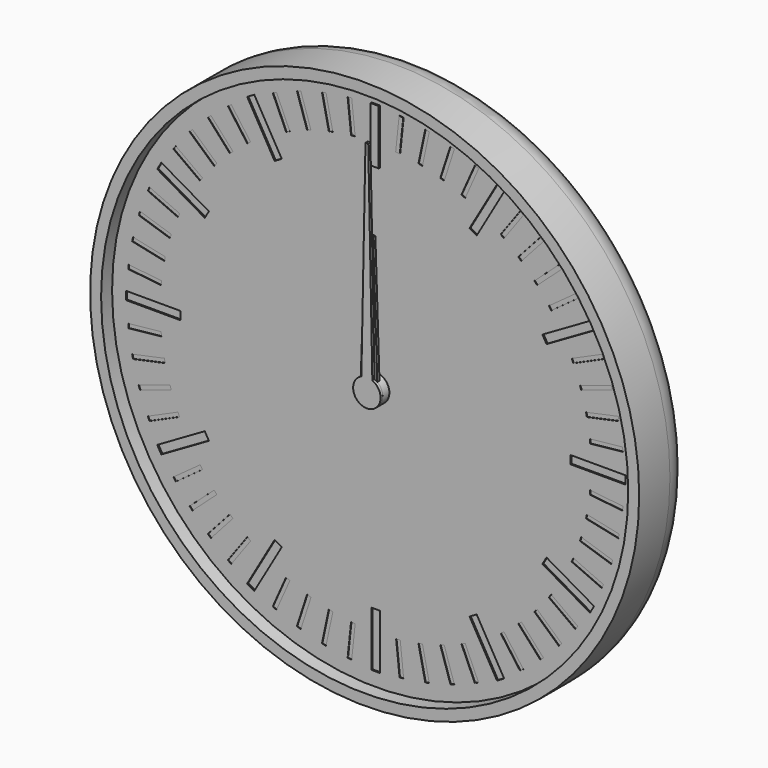
from build123d import *

# Parameters (mm, degrees)
F0_R      = 100
F1_DEPTH  = 24
F2_R      = 10
F3_T      = -4
F4_R      = 5
F4_R_2    = 3
F5_DEPTH  = 2
F6_DEPTH  = 19
F7_DEPTH  = 8
F9_DEPTH  = 4
F11_DEPTH = 4
F12_R     = 5
F12_R_2   = 3
F13_DEPTH = 2
F14_R     = 3
F15_DEPTH = 4
F17_DEPTH = 4
F18_R     = 3
F19_DEPTH = 2
F20_R     = 98
F20_R_2   = 5
F21_DEPTH = 1
F23_R     = 5
F23_R_2   = 3
F24_DEPTH = 2
F25_W     = 3
F25_H     = 20
F25_W_2   = 20
F25_H_2   = 3
F26_DEPTH = 0.5
F27_W     = 1.5
F27_H     = 12
F27_W_2   = 12
F27_H_2   = 1.5
F28_DEPTH = 0.2
F29_DEPTH = 1
F30_DEPTH = 0.4
F31_R     = 5
F31_R_2   = 3
F32_DEPTH = 5
F33_R     = 3
F34_DEPTH = 1
F36_DEPTH = 1


with BuildPart() as f1:
    # F0 (on Front) → F1 (new body)
    with BuildSketch(Plane.XZ):
        Circle(F0_R)
    extrude(amount=F1_DEPTH)

    # F2
    f2_edges = [f1.edges().sort_by_distance(p)[0] for p in [
        (-100, 0, 0),
    ]]
    fillet(f2_edges, radius=F2_R)

    # F3
    f3_openings = [f1.faces().sort_by_distance(p)[0] for p in [
        (0, -24, 0),
    ]]
    offset(amount=F3_T, openings=f3_openings)

    # F4 (on face) → F5 (join)
    with BuildSketch(Plane.XZ.offset(4)):
        Circle(F4_R)
        Circle(F4_R_2, mode=Mode.SUBTRACT)
        with Locations((40, 0)):
            Circle(F4_R)
        with Locations((40, 0)):
            Circle(F4_R_2, mode=Mode.SUBTRACT)
    extrude(amount=F5_DEPTH)


with BuildPart() as f6:
    # F6 (new): a face of the model
    f6_faces = [f1.part.faces().sort_by_distance(p)[0] for p in [
        (0, -4, 0),
    ]]
    extrude(f6_faces, amount=F6_DEPTH)

    # F8 (on face) → F9 (join)
    with BuildSketch(Plane.XZ.offset(6)):
        with BuildLine():
            ThreePointArc((9.2729637667, -1.3794085621), (9.3494561423, -0.6915886375), (9.375, 0))
            ThreePointArc((9.375, 0), (9.3494561423, 0.6915886375), (9.2729637667, 1.3794085621))
            ThreePointArc((9.2729637667, 1.3794085621), (8.9161548403, 2.8970343223), (8.3127812852, 4.3345463782))
            ThreePointArc((8.3127812852, 4.3345463782), (7.5845343223, 5.5104867402), (6.6911892658, 6.566476316))
            ThreePointArc((6.6911892658, 6.566476316), (5.5104867402, 7.5845343223), (4.1773988938, 8.3928519278))
            ThreePointArc((4.1773988938, 8.3928519278), (2.8970343223, 8.9161548403), (1.5536078905, 9.2453733036))
            ThreePointArc((1.5536078905, 9.2453733036), (0, 9.375), (-1.5536078905, 9.2453733036))
            ThreePointArc((-1.5536078905, 9.2453733036), (-2.8970343223, 8.9161548403), (-4.1773988938, 8.3928519278))
            ThreePointArc((-4.1773988938, 8.3928519278), (-5.5104867402, 7.5845343223), (-6.6911892658, 6.566476316))
            ThreePointArc((-6.6911892658, 6.566476316), (-7.5845343223, 5.5104867402), (-8.3127812852, 4.3345463782))
            ThreePointArc((-8.3127812852, 4.3345463782), (-8.9161548403, 2.8970343223), (-9.2729637667, 1.3794085621))
            ThreePointArc((-9.2729637667, 1.3794085621), (-9.375, 0), (-9.2729637667, -1.3794085621))
            ThreePointArc((-9.2729637667, -1.3794085621), (-8.9161548403, -2.8970343223), (-8.3127812852, -4.3345463782))
            ThreePointArc((-8.3127812852, -4.3345463782), (-7.5845343223, -5.5104867402), (-6.6911892658, -6.566476316))
            ThreePointArc((-6.6911892658, -6.566476316), (-5.5104867402, -7.5845343223), (-4.1773988938, -8.3928519278))
            ThreePointArc((-4.1773988938, -8.3928519278), (-2.8970343223, -8.9161548403), (-1.5536078905, -9.2453733036))
            ThreePointArc((-1.5536078905, -9.2453733036), (0, -9.375), (1.5536078905, -9.2453733036))
            ThreePointArc((1.5536078905, -9.2453733036), (2.8970343223, -8.9161548403), (4.1773988938, -8.3928519278))
            ThreePointArc((4.1773988938, -8.3928519278), (5.5104867402, -7.5845343223), (6.6911892658, -6.566476316))
            ThreePointArc((6.6911892658, -6.566476316), (7.5845343223, -5.5104867402), (8.3127812852, -4.3345463782))
            ThreePointArc((8.3127812852, -4.3345463782), (8.9161548403, -2.8970343223), (9.2729637667, -1.3794085621))
        make_face()
        with BuildLine():
            ThreePointArc((8.3127812852, 4.3345463782), (8.9161548403, 2.8970343223), (9.2729637667, 1.3794085621))
            Line((9.2729637667, 1.3794085621), (11.1823199426, 2.3946312492))
            Line((11.1823199426, 2.3946312492), (10.8182678729, 3.515068311))
            Line((10.8182678729, 3.515068311), (10.4542158031, 4.6355053728))
            Line((10.4542158031, 4.6355053728), (8.3127812852, 4.3345463782))
        make_face()
        with BuildLine():
            Line((11.1823199426, -2.3946312492), (9.2729637667, -1.3794085621))
            ThreePointArc((9.2729637667, -1.3794085621), (8.9161548403, -2.8970343223), (8.3127812852, -4.3345463782))
            Line((8.3127812852, -4.3345463782), (10.4542158031, -4.6355053728))
            Line((10.4542158031, -4.6355053728), (10.8182678729, -3.515068311))
            Line((10.8182678729, -3.515068311), (11.1823199426, -2.3946312492))
        make_face()
        with BuildLine():
            ThreePointArc((4.1773988938, 8.3928519278), (5.5104867402, 7.5845343223), (6.6911892658, 6.566476316))
            Line((6.6911892658, 6.566476316), (7.6391579371, 8.5101001246))
            Line((7.6391579371, 8.5101001246), (6.6860572448, 9.202568311))
            Line((6.6860572448, 9.202568311), (5.7329565525, 9.8950364974))
            Line((5.7329565525, 9.8950364974), (4.1773988938, 8.3928519278))
        make_face()
        with BuildLine():
            Line((7.6391579371, -8.5101001246), (6.6911892658, -6.566476316))
            ThreePointArc((6.6911892658, -6.566476316), (5.5104867402, -7.5845343223), (4.1773988938, -8.3928519278))
            Line((4.1773988938, -8.3928519278), (5.7329565525, -9.8950364974))
            Line((5.7329565525, -9.8950364974), (6.6860572448, -9.202568311))
            Line((6.6860572448, -9.202568311), (7.6391579371, -8.5101001246))
        make_face()
        with BuildLine():
            ThreePointArc((-1.5536078905, 9.2453733036), (0, 9.375), (1.5536078905, 9.2453733036))
            Line((1.5536078905, 9.2453733036), (1.1780972451, 11.375))
            Line((1.1780972451, 11.375), (0, 11.375))
            Line((0, 11.375), (-1.1780972451, 11.375))
            Line((-1.1780972451, 11.375), (-1.5536078905, 9.2453733036))
        make_face()
        with BuildLine():
            Line((1.1780972451, -11.375), (1.5536078905, -9.2453733036))
            ThreePointArc((1.5536078905, -9.2453733036), (0, -9.375), (-1.5536078905, -9.2453733036))
            Line((-1.5536078905, -9.2453733036), (-1.1780972451, -11.375))
            Line((-1.1780972451, -11.375), (0, -11.375))
            Line((0, -11.375), (1.1780972451, -11.375))
        make_face()
        with BuildLine():
            ThreePointArc((-6.6911892658, 6.566476316), (-5.5104867402, 7.5845343223), (-4.1773988938, 8.3928519278))
            Line((-4.1773988938, 8.3928519278), (-5.7329565525, 9.8950364974))
            Line((-5.7329565525, 9.8950364974), (-6.6860572448, 9.202568311))
            Line((-6.6860572448, 9.202568311), (-7.6391579371, 8.5101001246))
            Line((-7.6391579371, 8.5101001246), (-6.6911892658, 6.566476316))
        make_face()
        with BuildLine():
            Line((-5.7329565525, -9.8950364974), (-4.1773988938, -8.3928519278))
            ThreePointArc((-4.1773988938, -8.3928519278), (-5.5104867402, -7.5845343223), (-6.6911892658, -6.566476316))
            Line((-6.6911892658, -6.566476316), (-7.6391579371, -8.5101001246))
            Line((-7.6391579371, -8.5101001246), (-6.6860572448, -9.202568311))
            Line((-6.6860572448, -9.202568311), (-5.7329565525, -9.8950364974))
        make_face()
        with BuildLine():
            ThreePointArc((-9.2729637667, 1.3794085621), (-8.9161548403, 2.8970343223), (-8.3127812852, 4.3345463782))
            Line((-8.3127812852, 4.3345463782), (-10.4542158031, 4.6355053728))
            Line((-10.4542158031, 4.6355053728), (-10.8182678729, 3.515068311))
            Line((-10.8182678729, 3.515068311), (-11.1823199426, 2.3946312492))
            Line((-11.1823199426, 2.3946312492), (-9.2729637667, 1.3794085621))
        make_face()
        with BuildLine():
            Line((-10.4542158031, -4.6355053728), (-8.3127812852, -4.3345463782))
            ThreePointArc((-8.3127812852, -4.3345463782), (-8.9161548403, -2.8970343223), (-9.2729637667, -1.3794085621))
            Line((-9.2729637667, -1.3794085621), (-11.1823199426, -2.3946312492))
            Line((-11.1823199426, -2.3946312492), (-10.8182678729, -3.515068311))
            Line((-10.8182678729, -3.515068311), (-10.4542158031, -4.6355053728))
        make_face()
    extrude(amount=F9_DEPTH)

    # F35 (on face) → F36 (join)
    with BuildSketch(Plane.XZ.offset(23)):
        with BuildLine():
            ThreePointArc((-2, 4.582575695), (-2.7386127875, -4.1833001327), (5, 0))
            ThreePointArc((5, 0), (4.1833001327, 2.7386127875), (2, 4.582575695))
            ThreePointArc((2, 4.582575695), (0, 5), (-2, 4.582575695))
        make_face()
        with BuildLine():
            ThreePointArc((-2, 4.582575695), (0, 5), (2, 4.582575695))
            Line((2, 4.582575695), (0.5, 80))
            Line((0.5, 80), (0, 80))
            Line((0, 80), (-0.5, 80))
            Line((-0.5, 80), (-2, 4.582575695))
        make_face()
    extrude(amount=-F36_DEPTH)


with BuildPart() as f7:
    # F7 (new): a face of the model
    f7_faces = [f1.part.faces().sort_by_distance(p)[0] for p in [
        (40, -4, 0),
    ]]
    extrude(f7_faces, amount=F7_DEPTH)

    # F10 (on face) → F11 (join)
    with BuildSketch(Plane.XZ.offset(6)):
        with BuildLine():
            ThreePointArc((68.0829066802, -1.5381733945), (68.1144747006, -0.7693746225), (68.125, 0))
            ThreePointArc((68.125, 0), (68.1144747006, 0.7693746225), (68.0829066802, 1.5381733945))
            ThreePointArc((68.0829066802, 1.5381733945), (67.9709283072, 2.9398630294), (67.7890320221, 4.3342039956))
            ThreePointArc((67.7890320221, 4.3342039956), (67.5104012706, 5.8475163042), (67.1494235596, 7.3433252263))
            ThreePointArc((67.1494235596, 7.3433252263), (66.7484645208, 8.6911029668), (66.280643318, 10.0171558733))
            ThreePointArc((66.280643318, 10.0171558733), (65.6934659962, 11.4394680865), (65.0293803521, 12.8275385085))
            ThreePointArc((65.0293803521, 12.8275385085), (64.3569644814, 14.0625), (63.6236643925, 15.2623099717))
            ThreePointArc((63.6236643925, 15.2623099717), (62.7536029668, 16.5314602207), (61.815433119, 17.7511268046))
            ThreePointArc((61.815433119, 17.7511268046), (60.9009482166, 18.8192983038), (59.934217974, 19.8404278876))
            ThreePointArc((59.934217974, 19.8404278876), (58.8192983038, 20.9009482166), (57.6480467764, 21.8989056799))
            ThreePointArc((57.6480467764, 21.8989056799), (56.5314602207, 22.7536029668), (55.3735505752, 23.5514238999))
            ThreePointArc((55.3735505752, 23.5514238999), (54.0625, 24.3569644814), (52.709356105, 25.0895972944))
            ThreePointArc((52.709356105, 25.0895972944), (51.4394680865, 25.6934659962), (50.1409852457, 26.2331096755))
            ThreePointArc((50.1409852457, 26.2331096755), (48.6911029668, 26.7484645208), (47.2152055856, 27.1837531139))
            ThreePointArc((47.2152055856, 27.1837531139), (45.8475163042, 27.5104012706), (44.4652101991, 27.7682826779))
            ThreePointArc((44.4652101991, 27.7682826779), (42.9398630294, 27.9709283072), (41.4057159597, 28.0898484802))
            ThreePointArc((41.4057159597, 28.0898484802), (40, 28.125), (38.5942840403, 28.0898484802))
            ThreePointArc((38.5942840403, 28.0898484802), (37.0601369706, 27.9709283072), (35.5347898009, 27.7682826779))
            ThreePointArc((35.5347898009, 27.7682826779), (34.1524836958, 27.5104012706), (32.7847944144, 27.1837531139))
            ThreePointArc((32.7847944144, 27.1837531139), (31.3088970332, 26.7484645208), (29.8590147543, 26.2331096755))
            ThreePointArc((29.8590147543, 26.2331096755), (28.5605319135, 25.6934659962), (27.290643895, 25.0895972944))
            ThreePointArc((27.290643895, 25.0895972944), (25.9375, 24.3569644814), (24.6264494248, 23.5514238999))
            ThreePointArc((24.6264494248, 23.5514238999), (23.4685397793, 22.7536029668), (22.3519532236, 21.8989056799))
            ThreePointArc((22.3519532236, 21.8989056799), (21.1807016962, 20.9009482166), (20.065782026, 19.8404278876))
            ThreePointArc((20.065782026, 19.8404278876), (19.0990517834, 18.8192983038), (18.184566881, 17.7511268046))
            ThreePointArc((18.184566881, 17.7511268046), (17.2463970332, 16.5314602207), (16.3763356075, 15.2623099717))
            ThreePointArc((16.3763356075, 15.2623099717), (15.6430355186, 14.0625), (14.9706196479, 12.8275385085))
            ThreePointArc((14.9706196479, 12.8275385085), (14.3065340038, 11.4394680865), (13.719356682, 10.0171558733))
            ThreePointArc((13.719356682, 10.0171558733), (13.2515354792, 8.6911029668), (12.8505764404, 7.3433252263))
            ThreePointArc((12.8505764404, 7.3433252263), (12.4895987294, 5.8475163042), (12.2109679779, 4.3342039956))
            ThreePointArc((12.2109679779, 4.3342039956), (12.0290716928, 2.9398630294), (11.9170933198, 1.5381733945))
            ThreePointArc((11.9170933198, 1.5381733945), (11.875, 0), (11.9170933198, -1.5381733945))
            ThreePointArc((11.9170933198, -1.5381733945), (12.0290716928, -2.9398630294), (12.2109679779, -4.3342039956))
            ThreePointArc((12.2109679779, -4.3342039956), (12.4895987294, -5.8475163042), (12.8505764404, -7.3433252263))
            ThreePointArc((12.8505764404, -7.3433252263), (13.2515354792, -8.6911029668), (13.719356682, -10.0171558733))
            ThreePointArc((13.719356682, -10.0171558733), (14.3065340038, -11.4394680865), (14.9706196479, -12.8275385085))
            ThreePointArc((14.9706196479, -12.8275385085), (15.6430355186, -14.0625), (16.3763356075, -15.2623099717))
            ThreePointArc((16.3763356075, -15.2623099717), (17.2463970332, -16.5314602207), (18.184566881, -17.7511268046))
            ThreePointArc((18.184566881, -17.7511268046), (19.0990517834, -18.8192983038), (20.065782026, -19.8404278876))
            ThreePointArc((20.065782026, -19.8404278876), (21.1807016962, -20.9009482166), (22.3519532236, -21.8989056799))
            ThreePointArc((22.3519532236, -21.8989056799), (23.4685397793, -22.7536029668), (24.6264494248, -23.5514238999))
            ThreePointArc((24.6264494248, -23.5514238999), (25.9375, -24.3569644814), (27.290643895, -25.0895972944))
            ThreePointArc((27.290643895, -25.0895972944), (28.5605319135, -25.6934659962), (29.8590147543, -26.2331096755))
            ThreePointArc((29.8590147543, -26.2331096755), (31.3088970332, -26.7484645208), (32.7847944144, -27.1837531139))
            ThreePointArc((32.7847944144, -27.1837531139), (34.1524836958, -27.5104012706), (35.5347898009, -27.7682826779))
            ThreePointArc((35.5347898009, -27.7682826779), (37.0601369706, -27.9709283072), (38.5942840403, -28.0898484802))
            ThreePointArc((38.5942840403, -28.0898484802), (40, -28.125), (41.4057159597, -28.0898484802))
            ThreePointArc((41.4057159597, -28.0898484802), (42.9398630294, -27.9709283072), (44.4652101991, -27.7682826779))
            ThreePointArc((44.4652101991, -27.7682826779), (45.8475163042, -27.5104012706), (47.2152055856, -27.1837531139))
            ThreePointArc((47.2152055856, -27.1837531139), (48.6911029668, -26.7484645208), (50.1409852457, -26.2331096755))
            ThreePointArc((50.1409852457, -26.2331096755), (51.4394680865, -25.6934659962), (52.709356105, -25.0895972944))
            ThreePointArc((52.709356105, -25.0895972944), (54.0625, -24.3569644814), (55.3735505752, -23.5514238999))
            ThreePointArc((55.3735505752, -23.5514238999), (56.5314602207, -22.7536029668), (57.6480467764, -21.8989056799))
            ThreePointArc((57.6480467764, -21.8989056799), (58.8192983038, -20.9009482166), (59.934217974, -19.8404278876))
            ThreePointArc((59.934217974, -19.8404278876), (60.9009482166, -18.8192983038), (61.815433119, -17.7511268046))
            ThreePointArc((61.815433119, -17.7511268046), (62.7536029668, -16.5314602207), (63.6236643925, -15.2623099717))
            ThreePointArc((63.6236643925, -15.2623099717), (64.3569644814, -14.0625), (65.0293803521, -12.8275385085))
            ThreePointArc((65.0293803521, -12.8275385085), (65.6934659962, -11.4394680865), (66.280643318, -10.0171558733))
            ThreePointArc((66.280643318, -10.0171558733), (66.7484645208, -8.6911029668), (67.1494235596, -7.3433252263))
            ThreePointArc((67.1494235596, -7.3433252263), (67.5104012706, -5.8475163042), (67.7890320221, -4.3342039956))
            ThreePointArc((67.7890320221, -4.3342039956), (67.9709283072, -2.9398630294), (68.0829066802, -1.5381733945))
        make_face()
        with BuildLine():
            ThreePointArc((68.0829066802, 1.5381733945), (68.1144747006, 0.7693746225), (68.125, 0))
            ThreePointArc((68.125, 0), (68.1144747006, -0.7693746225), (68.0829066802, -1.5381733945))
            Line((68.0829066802, -1.5381733945), (70.125, -1.1780972451))
            Line((70.125, -1.1780972451), (70.125, 0))
            Line((70.125, 0), (70.125, 1.1780972451))
            Line((70.125, 1.1780972451), (68.0829066802, 1.5381733945))
        make_face()
        with BuildLine():
            ThreePointArc((67.1494235596, 7.3433252263), (67.5104012706, 5.8475163042), (67.7890320221, 4.3342039956))
            Line((67.7890320221, 4.3342039956), (69.7116366623, 5.1109866922))
            Line((69.7116366623, 5.1109866922), (69.4666964721, 6.2633396859))
            Line((69.4666964721, 6.2633396859), (69.2217562819, 7.4156926796))
            Line((69.2217562819, 7.4156926796), (67.1494235596, 7.3433252263))
        make_face()
        with BuildLine():
            Line((69.7116366623, -5.1109866922), (67.7890320221, -4.3342039956))
            ThreePointArc((67.7890320221, -4.3342039956), (67.5104012706, -5.8475163042), (67.1494235596, -7.3433252263))
            Line((67.1494235596, -7.3433252263), (69.2217562819, -7.4156926796))
            Line((69.2217562819, -7.4156926796), (69.4666964721, -6.2633396859))
            Line((69.4666964721, -6.2633396859), (69.7116366623, -5.1109866922))
        make_face()
        with BuildLine():
            ThreePointArc((65.0293803521, 12.8275385085), (65.6934659962, 11.4394680865), (66.280643318, 10.0171558733))
            Line((66.280643318, 10.0171558733), (67.9997322302, 11.1766959857))
            Line((67.9997322302, 11.1766959857), (67.5205569115, 12.2529413727))
            Line((67.5205569115, 12.2529413727), (67.0413815928, 13.3291867596))
            Line((67.0413815928, 13.3291867596), (65.0293803521, 12.8275385085))
        make_face()
        with BuildLine():
            Line((67.9997322302, -11.1766959857), (66.280643318, -10.0171558733))
            ThreePointArc((66.280643318, -10.0171558733), (65.6934659962, -11.4394680865), (65.0293803521, -12.8275385085))
            Line((65.0293803521, -12.8275385085), (67.0413815928, -13.3291867596))
            Line((67.0413815928, -13.3291867596), (67.5205569115, -12.2529413727))
            Line((67.5205569115, -12.2529413727), (67.9997322302, -11.1766959857))
        make_face()
        with BuildLine():
            ThreePointArc((61.815433119, 17.7511268046), (62.7536029668, 16.5314602207), (63.6236643925, 15.2623099717))
            Line((63.6236643925, 15.2623099717), (65.064105142, 16.753930033))
            Line((65.064105142, 16.753930033), (64.3716369555, 17.7070307253))
            Line((64.3716369555, 17.7070307253), (63.6791687691, 18.6601314176))
            Line((63.6791687691, 18.6601314176), (61.815433119, 17.7511268046))
        make_face()
        with BuildLine():
            Line((65.064105142, -16.753930033), (63.6236643925, -15.2623099717))
            ThreePointArc((63.6236643925, -15.2623099717), (62.7536029668, -16.5314602207), (61.815433119, -17.7511268046))
            Line((61.815433119, -17.7511268046), (63.6791687691, -18.6601314176))
            Line((63.6791687691, -18.6601314176), (64.3716369555, -17.7070307253))
            Line((64.3716369555, -17.7070307253), (65.064105142, -16.753930033))
        make_face()
        with BuildLine():
            ThreePointArc((57.6480467764, 21.8989056799), (58.8192983038, 20.9009482166), (59.934217974, 19.8404278876))
            Line((59.934217974, 19.8404278876), (61.0330563882, 21.5989369435))
            Line((61.0330563882, 21.5989369435), (60.1575595166, 22.3872378675))
            Line((60.1575595166, 22.3872378675), (59.282062645, 23.1755387915))
            Line((59.282062645, 23.1755387915), (57.6480467764, 21.8989056799))
        make_face()
        with BuildLine():
            Line((61.0330563882, -21.5989369435), (59.934217974, -19.8404278876))
            ThreePointArc((59.934217974, -19.8404278876), (58.8192983038, -20.9009482166), (57.6480467764, -21.8989056799))
            Line((57.6480467764, -21.8989056799), (59.282062645, -23.1755387915))
            Line((59.282062645, -23.1755387915), (60.1575595166, -22.3872378675))
            Line((60.1575595166, -22.3872378675), (61.0330563882, -21.5989369435))
        make_face()
        with BuildLine():
            ThreePointArc((52.709356105, 25.0895972944), (54.0625, 24.3569644814), (55.3735505752, 23.5514238999))
            Line((55.3735505752, 23.5514238999), (56.0827621424, 25.4999666665))
            Line((56.0827621424, 25.4999666665), (55.0625, 26.089015289))
            Line((55.0625, 26.089015289), (54.0422378576, 26.6780639116))
            Line((54.0422378576, 26.6780639116), (52.709356105, 25.0895972944))
        make_face()
        with BuildLine():
            Line((56.0827621424, -25.4999666665), (55.3735505752, -23.5514238999))
            ThreePointArc((55.3735505752, -23.5514238999), (54.0625, -24.3569644814), (52.709356105, -25.0895972944))
            Line((52.709356105, -25.0895972944), (54.0422378576, -26.6780639116))
            Line((54.0422378576, -26.6780639116), (55.0625, -26.089015289))
            Line((55.0625, -26.089015289), (56.0827621424, -25.4999666665))
        make_face()
        with BuildLine():
            ThreePointArc((47.2152055856, 27.1837531139), (48.6911029668, 26.7484645208), (50.1409852457, 26.2331096755))
            Line((50.1409852457, 26.2331096755), (50.4295740173, 28.2865254836))
            Line((50.4295740173, 28.2865254836), (49.3091369555, 28.6505775534))
            Line((49.3091369555, 28.6505775534), (48.1886998938, 29.0146296232))
            Line((48.1886998938, 29.0146296232), (47.2152055856, 27.1837531139))
        make_face()
        with BuildLine():
            Line((50.4295740173, -28.2865254836), (50.1409852457, -26.2331096755))
            ThreePointArc((50.1409852457, -26.2331096755), (48.6911029668, -26.7484645208), (47.2152055856, -27.1837531139))
            Line((47.2152055856, -27.1837531139), (48.1886998938, -29.0146296232))
            Line((48.1886998938, -29.0146296232), (49.3091369555, -28.6505775534))
            Line((49.3091369555, -28.6505775534), (50.4295740173, -28.2865254836))
        make_face()
        with BuildLine():
            ThreePointArc((41.4057159597, 28.0898484802), (42.9398630294, 27.9709283072), (44.4652101991, 27.7682826779))
            Line((44.4652101991, 27.7682826779), (44.3205634611, 29.8368274034))
            Line((44.3205634611, 29.8368274034), (43.1489199559, 29.959972098))
            Line((43.1489199559, 29.959972098), (41.9772764508, 30.0831167926))
            Line((41.9772764508, 30.0831167926), (41.4057159597, 28.0898484802))
        make_face()
        with BuildLine():
            Line((44.3205634611, -29.8368274034), (44.4652101991, -27.7682826779))
            ThreePointArc((44.4652101991, -27.7682826779), (42.9398630294, -27.9709283072), (41.4057159597, -28.0898484802))
            Line((41.4057159597, -28.0898484802), (41.9772764508, -30.0831167926))
            Line((41.9772764508, -30.0831167926), (43.1489199559, -29.959972098))
            Line((43.1489199559, -29.959972098), (44.3205634611, -29.8368274034))
        make_face()
        with BuildLine():
            ThreePointArc((35.5347898009, 27.7682826779), (37.0601369706, 27.9709283072), (38.5942840403, 28.0898484802))
            Line((38.5942840403, 28.0898484802), (38.0227235492, 30.0831167926))
            Line((38.0227235492, 30.0831167926), (36.8510800441, 29.959972098))
            Line((36.8510800441, 29.959972098), (35.6794365389, 29.8368274034))
            Line((35.6794365389, 29.8368274034), (35.5347898009, 27.7682826779))
        make_face()
        with BuildLine():
            Line((38.0227235492, -30.0831167926), (38.5942840403, -28.0898484802))
            ThreePointArc((38.5942840403, -28.0898484802), (37.0601369706, -27.9709283072), (35.5347898009, -27.7682826779))
            Line((35.5347898009, -27.7682826779), (35.6794365389, -29.8368274034))
            Line((35.6794365389, -29.8368274034), (36.8510800441, -29.959972098))
            Line((36.8510800441, -29.959972098), (38.0227235492, -30.0831167926))
        make_face()
        with BuildLine():
            ThreePointArc((29.8590147543, 26.2331096755), (31.3088970332, 26.7484645208), (32.7847944144, 27.1837531139))
            Line((32.7847944144, 27.1837531139), (31.8113001062, 29.0146296232))
            Line((31.8113001062, 29.0146296232), (30.6908630445, 28.6505775534))
            Line((30.6908630445, 28.6505775534), (29.5704259827, 28.2865254836))
            Line((29.5704259827, 28.2865254836), (29.8590147543, 26.2331096755))
        make_face()
        with BuildLine():
            Line((31.8113001062, -29.0146296232), (32.7847944144, -27.1837531139))
            ThreePointArc((32.7847944144, -27.1837531139), (31.3088970332, -26.7484645208), (29.8590147543, -26.2331096755))
            Line((29.8590147543, -26.2331096755), (29.5704259827, -28.2865254836))
            Line((29.5704259827, -28.2865254836), (30.6908630445, -28.6505775534))
            Line((30.6908630445, -28.6505775534), (31.8113001062, -29.0146296232))
        make_face()
        with BuildLine():
            ThreePointArc((24.6264494248, 23.5514238999), (25.9375, 24.3569644814), (27.290643895, 25.0895972944))
            Line((27.290643895, 25.0895972944), (25.9577621424, 26.6780639116))
            Line((25.9577621424, 26.6780639116), (24.9375, 26.089015289))
            Line((24.9375, 26.089015289), (23.9172378576, 25.4999666665))
            Line((23.9172378576, 25.4999666665), (24.6264494248, 23.5514238999))
        make_face()
        with BuildLine():
            Line((25.9577621424, -26.6780639116), (27.290643895, -25.0895972944))
            ThreePointArc((27.290643895, -25.0895972944), (25.9375, -24.3569644814), (24.6264494248, -23.5514238999))
            Line((24.6264494248, -23.5514238999), (23.9172378576, -25.4999666665))
            Line((23.9172378576, -25.4999666665), (24.9375, -26.089015289))
            Line((24.9375, -26.089015289), (25.9577621424, -26.6780639116))
        make_face()
        with BuildLine():
            ThreePointArc((20.065782026, 19.8404278876), (21.1807016962, 20.9009482166), (22.3519532236, 21.8989056799))
            Line((22.3519532236, 21.8989056799), (20.717937355, 23.1755387915))
            Line((20.717937355, 23.1755387915), (19.8424404834, 22.3872378675))
            Line((19.8424404834, 22.3872378675), (18.9669436118, 21.5989369435))
            Line((18.9669436118, 21.5989369435), (20.065782026, 19.8404278876))
        make_face()
        with BuildLine():
            Line((20.717937355, -23.1755387915), (22.3519532236, -21.8989056799))
            ThreePointArc((22.3519532236, -21.8989056799), (21.1807016962, -20.9009482166), (20.065782026, -19.8404278876))
            Line((20.065782026, -19.8404278876), (18.9669436118, -21.5989369435))
            Line((18.9669436118, -21.5989369435), (19.8424404834, -22.3872378675))
            Line((19.8424404834, -22.3872378675), (20.717937355, -23.1755387915))
        make_face()
        with BuildLine():
            ThreePointArc((16.3763356075, 15.2623099717), (17.2463970332, 16.5314602207), (18.184566881, 17.7511268046))
            Line((18.184566881, 17.7511268046), (16.3208312309, 18.6601314176))
            Line((16.3208312309, 18.6601314176), (15.6283630445, 17.7070307253))
            Line((15.6283630445, 17.7070307253), (14.935894858, 16.753930033))
            Line((14.935894858, 16.753930033), (16.3763356075, 15.2623099717))
        make_face()
        with BuildLine():
            Line((16.3208312309, -18.6601314176), (18.184566881, -17.7511268046))
            ThreePointArc((18.184566881, -17.7511268046), (17.2463970332, -16.5314602207), (16.3763356075, -15.2623099717))
            Line((16.3763356075, -15.2623099717), (14.935894858, -16.753930033))
            Line((14.935894858, -16.753930033), (15.6283630445, -17.7070307253))
            Line((15.6283630445, -17.7070307253), (16.3208312309, -18.6601314176))
        make_face()
        with BuildLine():
            ThreePointArc((13.719356682, 10.0171558733), (14.3065340038, 11.4394680865), (14.9706196479, 12.8275385085))
            Line((14.9706196479, 12.8275385085), (12.9586184072, 13.3291867596))
            Line((12.9586184072, 13.3291867596), (12.4794430885, 12.2529413727))
            Line((12.4794430885, 12.2529413727), (12.0002677698, 11.1766959857))
            Line((12.0002677698, 11.1766959857), (13.719356682, 10.0171558733))
        make_face()
        with BuildLine():
            Line((12.9586184072, -13.3291867596), (14.9706196479, -12.8275385085))
            ThreePointArc((14.9706196479, -12.8275385085), (14.3065340038, -11.4394680865), (13.719356682, -10.0171558733))
            Line((13.719356682, -10.0171558733), (12.0002677698, -11.1766959857))
            Line((12.0002677698, -11.1766959857), (12.4794430885, -12.2529413727))
            Line((12.4794430885, -12.2529413727), (12.9586184072, -13.3291867596))
        make_face()
        with BuildLine():
            ThreePointArc((12.2109679779, 4.3342039956), (12.4895987294, 5.8475163042), (12.8505764404, 7.3433252263))
            Line((12.8505764404, 7.3433252263), (10.7782437181, 7.4156926796))
            Line((10.7782437181, 7.4156926796), (10.5333035279, 6.2633396859))
            Line((10.5333035279, 6.2633396859), (10.2883633377, 5.1109866922))
            Line((10.2883633377, 5.1109866922), (12.2109679779, 4.3342039956))
        make_face()
        with BuildLine():
            Line((10.7782437181, -7.4156926796), (12.8505764404, -7.3433252263))
            ThreePointArc((12.8505764404, -7.3433252263), (12.4895987294, -5.8475163042), (12.2109679779, -4.3342039956))
            Line((12.2109679779, -4.3342039956), (10.2883633377, -5.1109866922))
            Line((10.2883633377, -5.1109866922), (10.5333035279, -6.2633396859))
            Line((10.5333035279, -6.2633396859), (10.7782437181, -7.4156926796))
        make_face()
        with BuildLine():
            ThreePointArc((11.9170933198, -1.5381733945), (11.875, 0), (11.9170933198, 1.5381733945))
            Line((11.9170933198, 1.5381733945), (9.875, 1.1780972451))
            Line((9.875, 1.1780972451), (9.875, 0))
            Line((9.875, 0), (9.875, -1.1780972451))
            Line((9.875, -1.1780972451), (11.9170933198, -1.5381733945))
        make_face()
    extrude(amount=F11_DEPTH)

    # F16 (on face) → F17 (join)
    with BuildSketch(Plane.XZ.offset(12)):
        with BuildLine():
            ThreePointArc((47.4288750323, -1.0304444454), (47.4821976298, -0.5164480894), (47.5, 0))
            ThreePointArc((47.5, 0), (47.4821976298, 0.5164480894), (47.4288750323, 1.0304444454))
            ThreePointArc((47.4288750323, 1.0304444454), (47.1329238722, 2.3176274578), (46.6157661985, 3.532936117))
            ThreePointArc((46.6157661985, 3.532936117), (46.0676274578, 4.4083893922), (45.4044061018, 5.2002302532))
            ThreePointArc((45.4044061018, 5.2002302532), (44.4083893922, 6.0676274578), (43.2756595386, 6.7468551628))
            ThreePointArc((43.2756595386, 6.7468551628), (42.3176274578, 7.1329238722), (41.3156377295, 7.3837048536))
            ThreePointArc((41.3156377295, 7.3837048536), (40, 7.5), (38.6843622705, 7.3837048536))
            ThreePointArc((38.6843622705, 7.3837048536), (37.6823725422, 7.1329238722), (36.7243404614, 6.7468551628))
            ThreePointArc((36.7243404614, 6.7468551628), (35.5916106078, 6.0676274578), (34.5955938982, 5.2002302532))
            ThreePointArc((34.5955938982, 5.2002302532), (33.9323725422, 4.4083893922), (33.3842338015, 3.532936117))
            ThreePointArc((33.3842338015, 3.532936117), (32.8670761278, 2.3176274578), (32.5711249677, 1.0304444454))
            ThreePointArc((32.5711249677, 1.0304444454), (32.5, 0), (32.5711249677, -1.0304444454))
            ThreePointArc((32.5711249677, -1.0304444454), (32.8670761278, -2.3176274578), (33.3842338015, -3.532936117))
            ThreePointArc((33.3842338015, -3.532936117), (33.9323725422, -4.4083893922), (34.5955938982, -5.2002302532))
            ThreePointArc((34.5955938982, -5.2002302532), (35.5916106078, -6.0676274578), (36.7243404614, -6.7468551628))
            ThreePointArc((36.7243404614, -6.7468551628), (37.6823725422, -7.1329238722), (38.6843622705, -7.3837048536))
            ThreePointArc((38.6843622705, -7.3837048536), (40, -7.5), (41.3156377295, -7.3837048536))
            ThreePointArc((41.3156377295, -7.3837048536), (42.3176274578, -7.1329238722), (43.2756595386, -6.7468551628))
            ThreePointArc((43.2756595386, -6.7468551628), (44.4083893922, -6.0676274578), (45.4044061018, -5.2002302532))
            ThreePointArc((45.4044061018, -5.2002302532), (46.0676274578, -4.4083893922), (46.6157661985, -3.532936117))
            ThreePointArc((46.6157661985, -3.532936117), (47.1329238722, -2.3176274578), (47.4288750323, -1.0304444454))
        make_face()
        with BuildLine():
            ThreePointArc((46.6157661985, 3.532936117), (47.1329238722, 2.3176274578), (47.4288750323, 1.0304444454))
            Line((47.4288750323, 1.0304444454), (49.3262785606, 2.0393117971))
            Line((49.3262785606, 2.0393117971), (48.743795249, 3.832011096))
            Line((48.743795249, 3.832011096), (46.6157661985, 3.532936117))
        make_face()
        with BuildLine():
            Line((49.3262785606, -2.0393117971), (47.4288750323, -1.0304444454))
            ThreePointArc((47.4288750323, -1.0304444454), (47.1329238722, -2.3176274578), (46.6157661985, -3.532936117))
            Line((46.6157661985, -3.532936117), (48.743795249, -3.832011096))
            Line((48.743795249, -3.832011096), (49.3262785606, -2.0393117971))
        make_face()
        with BuildLine():
            ThreePointArc((43.2756595386, 6.7468551628), (44.4083893922, 6.0676274578), (45.4044061018, 5.2002302532))
            Line((45.4044061018, 5.2002302532), (46.3464404506, 7.1316868974))
            Line((46.3464404506, 7.1316868974), (44.8214793429, 8.2396359957))
            Line((44.8214793429, 8.2396359957), (43.2756595386, 6.7468551628))
        make_face()
        with BuildLine():
            Line((46.3464404506, -7.1316868974), (45.4044061018, -5.2002302532))
            ThreePointArc((45.4044061018, -5.2002302532), (44.4083893922, -6.0676274578), (43.2756595386, -6.7468551628))
            Line((43.2756595386, -6.7468551628), (44.8214793429, -8.2396359957))
            Line((44.8214793429, -8.2396359957), (46.3464404506, -7.1316868974))
        make_face()
        with BuildLine():
            ThreePointArc((38.6843622705, 7.3837048536), (40, 7.5), (41.3156377295, 7.3837048536))
            Line((41.3156377295, 7.3837048536), (40.9424777961, 9.5))
            Line((40.9424777961, 9.5), (39.0575222039, 9.5))
            Line((39.0575222039, 9.5), (38.6843622705, 7.3837048536))
        make_face()
        with BuildLine():
            Line((40.9424777961, -9.5), (41.3156377295, -7.3837048536))
            ThreePointArc((41.3156377295, -7.3837048536), (40, -7.5), (38.6843622705, -7.3837048536))
            Line((38.6843622705, -7.3837048536), (39.0575222039, -9.5))
            Line((39.0575222039, -9.5), (40.9424777961, -9.5))
        make_face()
        with BuildLine():
            ThreePointArc((34.5955938982, 5.2002302532), (35.5916106078, 6.0676274578), (36.7243404614, 6.7468551628))
            Line((36.7243404614, 6.7468551628), (35.1785206571, 8.2396359957))
            Line((35.1785206571, 8.2396359957), (33.6535595494, 7.1316868974))
            Line((33.6535595494, 7.1316868974), (34.5955938982, 5.2002302532))
        make_face()
        with BuildLine():
            Line((35.1785206571, -8.2396359957), (36.7243404614, -6.7468551628))
            ThreePointArc((36.7243404614, -6.7468551628), (35.5916106078, -6.0676274578), (34.5955938982, -5.2002302532))
            Line((34.5955938982, -5.2002302532), (33.6535595494, -7.1316868974))
            Line((33.6535595494, -7.1316868974), (35.1785206571, -8.2396359957))
        make_face()
        with BuildLine():
            ThreePointArc((32.5711249677, 1.0304444454), (32.8670761278, 2.3176274578), (33.3842338015, 3.532936117))
            Line((33.3842338015, 3.532936117), (31.256204751, 3.832011096))
            Line((31.256204751, 3.832011096), (30.6737214394, 2.0393117971))
            Line((30.6737214394, 2.0393117971), (32.5711249677, 1.0304444454))
        make_face()
        with BuildLine():
            Line((31.256204751, -3.832011096), (33.3842338015, -3.532936117))
            ThreePointArc((33.3842338015, -3.532936117), (32.8670761278, -2.3176274578), (32.5711249677, -1.0304444454))
            Line((32.5711249677, -1.0304444454), (30.6737214394, -2.0393117971))
            Line((30.6737214394, -2.0393117971), (31.256204751, -3.832011096))
        make_face()
    extrude(amount=F17_DEPTH)

    # F18 (on face) → F19 (join)
    with BuildSketch(Plane.XZ.offset(16)):
        with Locations((40, 0)):
            Circle(F18_R)
    extrude(amount=F19_DEPTH)


with BuildPart() as f13:
    # F12 (on face) → F13 (new body)
    with BuildSketch(Plane.XZ.offset(10)):
        Circle(F12_R)
        Circle(F12_R_2, mode=Mode.SUBTRACT)
    extrude(amount=F13_DEPTH)

    # F14 (on face) → F15 (join)
    with BuildSketch(Plane.XZ.offset(12)):
        with BuildLine():
            ThreePointArc((29.9718156995, -1.3001014101), (29.9929530972, -0.6502034357), (30, 0))
            ThreePointArc((30, 0), (29.9929530972, 0.6502034357), (29.9718156995, 1.3001014101))
            ThreePointArc((29.9718156995, 1.3001014101), (29.907520012, 2.3537728718), (29.8061935814, 3.4045299509))
            ThreePointArc((29.8061935814, 3.4045299509), (29.6306502179, 4.6930339512), (29.3994322443, 5.9727199596))
            ThreePointArc((29.3994322443, 5.9727199596), (29.1710976119, 7.0033609157), (28.9066440563, 8.0253304855))
            ThreePointArc((28.9066440563, 8.0253304855), (28.5316954889, 9.2705098312), (28.1031371961, 10.4982703213))
            ThreePointArc((28.1031371961, 10.4982703213), (27.7163859753, 11.480502971), (27.2953170189, 12.448520749))
            ThreePointArc((27.2953170189, 12.448520749), (26.7301957257, 13.6197149922), (26.1148496411, 14.765318426))
            ThreePointArc((26.1148496411, 14.765318426), (25.5792049306, 15.6749569415), (25.0118886885, 16.5651871174))
            ThreePointArc((25.0118886885, 16.5651871174), (24.2705098312, 17.6335575688), (23.4835278178, 18.6687953878))
            ThreePointArc((23.4835278178, 18.6687953878), (22.812178968, 19.4834414499), (22.1125846489, 20.2739636023))
            ThreePointArc((22.1125846489, 20.2739636023), (21.2132034356, 21.2132034356), (20.2739636023, 22.1125846489))
            ThreePointArc((20.2739636023, 22.1125846489), (19.4834414499, 22.812178968), (18.6687953878, 23.4835278178))
            ThreePointArc((18.6687953878, 23.4835278178), (17.6335575688, 24.2705098312), (16.5651871174, 25.0118886885))
            ThreePointArc((16.5651871174, 25.0118886885), (15.6749569415, 25.5792049306), (14.765318426, 26.1148496411))
            ThreePointArc((14.765318426, 26.1148496411), (13.6197149922, 26.7301957257), (12.448520749, 27.2953170189))
            ThreePointArc((12.448520749, 27.2953170189), (11.480502971, 27.7163859753), (10.4982703213, 28.1031371961))
            ThreePointArc((10.4982703213, 28.1031371961), (9.2705098312, 28.5316954889), (8.0253304855, 28.9066440563))
            ThreePointArc((8.0253304855, 28.9066440563), (7.0033609157, 29.1710976119), (5.9727199596, 29.3994322443))
            ThreePointArc((5.9727199596, 29.3994322443), (4.6930339512, 29.6306502179), (3.4045299509, 29.8061935814))
            ThreePointArc((3.4045299509, 29.8061935814), (2.3537728718, 29.907520012), (1.3001014101, 29.9718156995))
            ThreePointArc((1.3001014101, 29.9718156995), (0, 30), (-1.3001014101, 29.9718156995))
            ThreePointArc((-1.3001014101, 29.9718156995), (-2.3537728718, 29.907520012), (-3.4045299509, 29.8061935814))
            ThreePointArc((-3.4045299509, 29.8061935814), (-4.6930339512, 29.6306502179), (-5.9727199596, 29.3994322443))
            ThreePointArc((-5.9727199596, 29.3994322443), (-7.0033609157, 29.1710976119), (-8.0253304855, 28.9066440563))
            ThreePointArc((-8.0253304855, 28.9066440563), (-9.2705098312, 28.5316954889), (-10.4982703213, 28.1031371961))
            ThreePointArc((-10.4982703213, 28.1031371961), (-11.480502971, 27.7163859753), (-12.448520749, 27.2953170189))
            ThreePointArc((-12.448520749, 27.2953170189), (-13.6197149922, 26.7301957257), (-14.765318426, 26.1148496411))
            ThreePointArc((-14.765318426, 26.1148496411), (-15.6749569415, 25.5792049306), (-16.5651871174, 25.0118886885))
            ThreePointArc((-16.5651871174, 25.0118886885), (-17.6335575688, 24.2705098312), (-18.6687953878, 23.4835278178))
            ThreePointArc((-18.6687953878, 23.4835278178), (-19.4834414499, 22.812178968), (-20.2739636023, 22.1125846489))
            ThreePointArc((-20.2739636023, 22.1125846489), (-21.2132034356, 21.2132034356), (-22.1125846489, 20.2739636023))
            ThreePointArc((-22.1125846489, 20.2739636023), (-22.812178968, 19.4834414499), (-23.4835278178, 18.6687953878))
            ThreePointArc((-23.4835278178, 18.6687953878), (-24.2705098312, 17.6335575688), (-25.0118886885, 16.5651871174))
            ThreePointArc((-25.0118886885, 16.5651871174), (-25.5792049306, 15.6749569415), (-26.1148496411, 14.765318426))
            ThreePointArc((-26.1148496411, 14.765318426), (-26.7301957257, 13.6197149922), (-27.2953170189, 12.448520749))
            ThreePointArc((-27.2953170189, 12.448520749), (-27.7163859753, 11.480502971), (-28.1031371961, 10.4982703213))
            ThreePointArc((-28.1031371961, 10.4982703213), (-28.5316954889, 9.2705098312), (-28.9066440563, 8.0253304855))
            ThreePointArc((-28.9066440563, 8.0253304855), (-29.1710976119, 7.0033609157), (-29.3994322443, 5.9727199596))
            ThreePointArc((-29.3994322443, 5.9727199596), (-29.6306502179, 4.6930339512), (-29.8061935814, 3.4045299509))
            ThreePointArc((-29.8061935814, 3.4045299509), (-29.907520012, 2.3537728718), (-29.9718156995, 1.3001014101))
            ThreePointArc((-29.9718156995, 1.3001014101), (-30, 0), (-29.9718156995, -1.3001014101))
            ThreePointArc((-29.9718156995, -1.3001014101), (-29.907520012, -2.3537728718), (-29.8061935814, -3.4045299509))
            ThreePointArc((-29.8061935814, -3.4045299509), (-29.6306502179, -4.6930339512), (-29.3994322443, -5.9727199596))
            ThreePointArc((-29.3994322443, -5.9727199596), (-29.1710976119, -7.0033609157), (-28.9066440563, -8.0253304855))
            ThreePointArc((-28.9066440563, -8.0253304855), (-28.5316954889, -9.2705098312), (-28.1031371961, -10.4982703213))
            ThreePointArc((-28.1031371961, -10.4982703213), (-27.7163859753, -11.480502971), (-27.2953170189, -12.448520749))
            ThreePointArc((-27.2953170189, -12.448520749), (-26.7301957257, -13.6197149922), (-26.1148496411, -14.765318426))
            ThreePointArc((-26.1148496411, -14.765318426), (-25.5792049306, -15.6749569415), (-25.0118886885, -16.5651871174))
            ThreePointArc((-25.0118886885, -16.5651871174), (-24.2705098312, -17.6335575688), (-23.4835278178, -18.6687953878))
            ThreePointArc((-23.4835278178, -18.6687953878), (-22.812178968, -19.4834414499), (-22.1125846489, -20.2739636023))
            ThreePointArc((-22.1125846489, -20.2739636023), (-21.2132034356, -21.2132034356), (-20.2739636023, -22.1125846489))
            ThreePointArc((-20.2739636023, -22.1125846489), (-19.4834414499, -22.812178968), (-18.6687953878, -23.4835278178))
            ThreePointArc((-18.6687953878, -23.4835278178), (-17.6335575688, -24.2705098312), (-16.5651871174, -25.0118886885))
            ThreePointArc((-16.5651871174, -25.0118886885), (-15.6749569415, -25.5792049306), (-14.765318426, -26.1148496411))
            ThreePointArc((-14.765318426, -26.1148496411), (-13.6197149922, -26.7301957257), (-12.448520749, -27.2953170189))
            ThreePointArc((-12.448520749, -27.2953170189), (-11.480502971, -27.7163859753), (-10.4982703213, -28.1031371961))
            ThreePointArc((-10.4982703213, -28.1031371961), (-9.2705098312, -28.5316954889), (-8.0253304855, -28.9066440563))
            ThreePointArc((-8.0253304855, -28.9066440563), (-7.0033609157, -29.1710976119), (-5.9727199596, -29.3994322443))
            ThreePointArc((-5.9727199596, -29.3994322443), (-4.6930339512, -29.6306502179), (-3.4045299509, -29.8061935814))
            ThreePointArc((-3.4045299509, -29.8061935814), (-2.3537728718, -29.907520012), (-1.3001014101, -29.9718156995))
            ThreePointArc((-1.3001014101, -29.9718156995), (0, -30), (1.3001014101, -29.9718156995))
            ThreePointArc((1.3001014101, -29.9718156995), (2.3537728718, -29.907520012), (3.4045299509, -29.8061935814))
            ThreePointArc((3.4045299509, -29.8061935814), (4.6930339512, -29.6306502179), (5.9727199596, -29.3994322443))
            ThreePointArc((5.9727199596, -29.3994322443), (7.0033609157, -29.1710976119), (8.0253304855, -28.9066440563))
            ThreePointArc((8.0253304855, -28.9066440563), (9.2705098312, -28.5316954889), (10.4982703213, -28.1031371961))
            ThreePointArc((10.4982703213, -28.1031371961), (11.480502971, -27.7163859753), (12.448520749, -27.2953170189))
            ThreePointArc((12.448520749, -27.2953170189), (13.6197149922, -26.7301957257), (14.765318426, -26.1148496411))
            ThreePointArc((14.765318426, -26.1148496411), (15.6749569415, -25.5792049306), (16.5651871174, -25.0118886885))
            ThreePointArc((16.5651871174, -25.0118886885), (17.6335575688, -24.2705098312), (18.6687953878, -23.4835278178))
            ThreePointArc((18.6687953878, -23.4835278178), (19.4834414499, -22.812178968), (20.2739636023, -22.1125846489))
            ThreePointArc((20.2739636023, -22.1125846489), (21.2132034356, -21.2132034356), (22.1125846489, -20.2739636023))
            ThreePointArc((22.1125846489, -20.2739636023), (22.812178968, -19.4834414499), (23.4835278178, -18.6687953878))
            ThreePointArc((23.4835278178, -18.6687953878), (24.2705098312, -17.6335575688), (25.0118886885, -16.5651871174))
            ThreePointArc((25.0118886885, -16.5651871174), (25.5792049306, -15.6749569415), (26.1148496411, -14.765318426))
            ThreePointArc((26.1148496411, -14.765318426), (26.7301957257, -13.6197149922), (27.2953170189, -12.448520749))
            ThreePointArc((27.2953170189, -12.448520749), (27.7163859753, -11.480502971), (28.1031371961, -10.4982703213))
            ThreePointArc((28.1031371961, -10.4982703213), (28.5316954889, -9.2705098312), (28.9066440563, -8.0253304855))
            ThreePointArc((28.9066440563, -8.0253304855), (29.1710976119, -7.0033609157), (29.3994322443, -5.9727199596))
            ThreePointArc((29.3994322443, -5.9727199596), (29.6306502179, -4.6930339512), (29.8061935814, -3.4045299509))
            ThreePointArc((29.8061935814, -3.4045299509), (29.907520012, -2.3537728718), (29.9718156995, -1.3001014101))
        make_face()
        Circle(F14_R, mode=Mode.SUBTRACT)
        with BuildLine():
            ThreePointArc((29.9718156995, 1.3001014101), (29.9929530972, 0.6502034357), (30, 0))
            ThreePointArc((30, 0), (29.9929530972, -0.6502034357), (29.9718156995, -1.3001014101))
            Line((29.9718156995, -1.3001014101), (32, -0.9424777961))
            Line((32, -0.9424777961), (32, 0))
            Line((32, 0), (32, 0.9424777961))
            Line((32, 0.9424777961), (29.9718156995, 1.3001014101))
        make_face()
        with BuildLine():
            ThreePointArc((29.3994322443, 5.9727199596), (29.6306502179, 4.6930339512), (29.8061935814, 3.4045299509))
            Line((29.8061935814, 3.4045299509), (31.7534629089, 4.0750285508))
            Line((31.7534629089, 4.0750285508), (31.606026899, 5.0059028813))
            Line((31.606026899, 5.0059028813), (31.4585908892, 5.9367772117))
            Line((31.4585908892, 5.9367772117), (29.3994322443, 5.9727199596))
        make_face()
        with BuildLine():
            Line((31.7534629089, -4.0750285508), (29.8061935814, -3.4045299509))
            ThreePointArc((29.8061935814, -3.4045299509), (29.6306502179, -4.6930339512), (29.3994322443, -5.9727199596))
            Line((29.3994322443, -5.9727199596), (31.4585908892, -5.9367772117))
            Line((31.4585908892, -5.9367772117), (31.606026899, -5.0059028813))
            Line((31.606026899, -5.0059028813), (31.7534629089, -4.0750285508))
        make_face()
        with BuildLine():
            ThreePointArc((28.1031371961, 10.4982703213), (28.5316954889, 9.2705098312), (28.9066440563, 8.0253304855))
            Line((28.9066440563, 8.0253304855), (30.7250501773, 8.9921941706))
            Line((30.7250501773, 8.9921941706), (30.4338085214, 9.88854382))
            Line((30.4338085214, 9.88854382), (30.1425668656, 10.7848934694))
            Line((30.1425668656, 10.7848934694), (28.1031371961, 10.4982703213))
        make_face()
        with BuildLine():
            Line((30.7250501773, -8.9921941706), (28.9066440563, -8.0253304855))
            ThreePointArc((28.9066440563, -8.0253304855), (28.5316954889, -9.2705098312), (28.1031371961, -10.4982703213))
            Line((28.1031371961, -10.4982703213), (30.1425668656, -10.7848934694))
            Line((30.1425668656, -10.7848934694), (30.4338085214, -9.88854382))
            Line((30.4338085214, -9.88854382), (30.7250501773, -8.9921941706))
        make_face()
        with BuildLine():
            ThreePointArc((26.1148496411, 14.765318426), (26.7301957257, 13.6197149922), (27.2953170189, 12.448520749))
            Line((27.2953170189, 12.448520749), (28.9400847397, 13.6879421265))
            Line((28.9400847397, 13.6879421265), (28.512208774, 14.5276959917))
            Line((28.512208774, 14.5276959917), (28.0843328084, 15.3674498569))
            Line((28.0843328084, 15.3674498569), (26.1148496411, 14.765318426))
        make_face()
        with BuildLine():
            Line((28.9400847397, -13.6879421265), (27.2953170189, -12.448520749))
            ThreePointArc((27.2953170189, -12.448520749), (26.7301957257, -13.6197149922), (26.1148496411, -14.765318426))
            Line((26.1148496411, -14.765318426), (28.0843328084, -15.3674498569))
            Line((28.0843328084, -15.3674498569), (28.512208774, -14.5276959917))
            Line((28.512208774, -14.5276959917), (28.9400847397, -13.6879421265))
        make_face()
        with BuildLine():
            ThreePointArc((23.4835278178, 18.6687953878), (24.2705098312, 17.6335575688), (25.0118886885, 16.5651871174))
            Line((25.0118886885, 16.5651871174), (26.4425183691, 18.0466475195))
            Line((26.4425183691, 18.0466475195), (25.88854382, 18.8091280734))
            Line((25.88854382, 18.8091280734), (25.3345692709, 19.5716086272))
            Line((25.3345692709, 19.5716086272), (23.4835278178, 18.6687953878))
        make_face()
        with BuildLine():
            Line((26.4425183691, -18.0466475195), (25.0118886885, -16.5651871174))
            ThreePointArc((25.0118886885, -16.5651871174), (24.2705098312, -17.6335575688), (23.4835278178, -18.6687953878))
            Line((23.4835278178, -18.6687953878), (25.3345692709, -19.5716086272))
            Line((25.3345692709, -19.5716086272), (25.88854382, -18.8091280734))
            Line((25.88854382, -18.8091280734), (26.4425183691, -18.0466475195))
        make_face()
        with BuildLine():
            ThreePointArc((20.2739636023, 22.1125846489), (21.2132034356, 21.2132034356), (22.1125846489, 20.2739636023))
            Line((22.1125846489, 20.2739636023), (23.2938494387, 21.9609845572))
            Line((23.2938494387, 21.9609845572), (22.627416998, 22.627416998))
            Line((22.627416998, 22.627416998), (21.9609845572, 23.2938494387))
            Line((21.9609845572, 23.2938494387), (20.2739636023, 22.1125846489))
        make_face()
        with BuildLine():
            Line((23.2938494387, -21.9609845572), (22.1125846489, -20.2739636023))
            ThreePointArc((22.1125846489, -20.2739636023), (21.2132034356, -21.2132034356), (20.2739636023, -22.1125846489))
            Line((20.2739636023, -22.1125846489), (21.9609845572, -23.2938494387))
            Line((21.9609845572, -23.2938494387), (22.627416998, -22.627416998))
            Line((22.627416998, -22.627416998), (23.2938494387, -21.9609845572))
        make_face()
        with BuildLine():
            ThreePointArc((16.5651871174, 25.0118886885), (17.6335575688, 24.2705098312), (18.6687953878, 23.4835278178))
            Line((18.6687953878, 23.4835278178), (19.5716086272, 25.3345692709))
            Line((19.5716086272, 25.3345692709), (18.8091280734, 25.88854382))
            Line((18.8091280734, 25.88854382), (18.0466475195, 26.4425183691))
            Line((18.0466475195, 26.4425183691), (16.5651871174, 25.0118886885))
        make_face()
        with BuildLine():
            Line((19.5716086272, -25.3345692709), (18.6687953878, -23.4835278178))
            ThreePointArc((18.6687953878, -23.4835278178), (17.6335575688, -24.2705098312), (16.5651871174, -25.0118886885))
            Line((16.5651871174, -25.0118886885), (18.0466475195, -26.4425183691))
            Line((18.0466475195, -26.4425183691), (18.8091280734, -25.88854382))
            Line((18.8091280734, -25.88854382), (19.5716086272, -25.3345692709))
        make_face()
        with BuildLine():
            ThreePointArc((12.448520749, 27.2953170189), (13.6197149922, 26.7301957257), (14.765318426, 26.1148496411))
            Line((14.765318426, 26.1148496411), (15.3674498569, 28.0843328084))
            Line((15.3674498569, 28.0843328084), (14.5276959917, 28.512208774))
            Line((14.5276959917, 28.512208774), (13.6879421265, 28.9400847397))
            Line((13.6879421265, 28.9400847397), (12.448520749, 27.2953170189))
        make_face()
        with BuildLine():
            Line((15.3674498569, -28.0843328084), (14.765318426, -26.1148496411))
            ThreePointArc((14.765318426, -26.1148496411), (13.6197149922, -26.7301957257), (12.448520749, -27.2953170189))
            Line((12.448520749, -27.2953170189), (13.6879421265, -28.9400847397))
            Line((13.6879421265, -28.9400847397), (14.5276959917, -28.512208774))
            Line((14.5276959917, -28.512208774), (15.3674498569, -28.0843328084))
        make_face()
        with BuildLine():
            ThreePointArc((8.0253304855, 28.9066440563), (9.2705098312, 28.5316954889), (10.4982703213, 28.1031371961))
            Line((10.4982703213, 28.1031371961), (10.7848934694, 30.1425668656))
            Line((10.7848934694, 30.1425668656), (9.88854382, 30.4338085214))
            Line((9.88854382, 30.4338085214), (8.9921941706, 30.7250501773))
            Line((8.9921941706, 30.7250501773), (8.0253304855, 28.9066440563))
        make_face()
        with BuildLine():
            Line((10.7848934694, -30.1425668656), (10.4982703213, -28.1031371961))
            ThreePointArc((10.4982703213, -28.1031371961), (9.2705098312, -28.5316954889), (8.0253304855, -28.9066440563))
            Line((8.0253304855, -28.9066440563), (8.9921941706, -30.7250501773))
            Line((8.9921941706, -30.7250501773), (9.88854382, -30.4338085214))
            Line((9.88854382, -30.4338085214), (10.7848934694, -30.1425668656))
        make_face()
        with BuildLine():
            ThreePointArc((3.4045299509, 29.8061935814), (4.6930339512, 29.6306502179), (5.9727199596, 29.3994322443))
            Line((5.9727199596, 29.3994322443), (5.9367772117, 31.4585908892))
            Line((5.9367772117, 31.4585908892), (5.0059028813, 31.606026899))
            Line((5.0059028813, 31.606026899), (4.0750285508, 31.7534629089))
            Line((4.0750285508, 31.7534629089), (3.4045299509, 29.8061935814))
        make_face()
        with BuildLine():
            Line((5.9367772117, -31.4585908892), (5.9727199596, -29.3994322443))
            ThreePointArc((5.9727199596, -29.3994322443), (4.6930339512, -29.6306502179), (3.4045299509, -29.8061935814))
            Line((3.4045299509, -29.8061935814), (4.0750285508, -31.7534629089))
            Line((4.0750285508, -31.7534629089), (5.0059028813, -31.606026899))
            Line((5.0059028813, -31.606026899), (5.9367772117, -31.4585908892))
        make_face()
        with BuildLine():
            ThreePointArc((-1.3001014101, 29.9718156995), (0, 30), (1.3001014101, 29.9718156995))
            Line((1.3001014101, 29.9718156995), (0.9424777961, 32))
            Line((0.9424777961, 32), (0, 32))
            Line((0, 32), (-0.9424777961, 32))
            Line((-0.9424777961, 32), (-1.3001014101, 29.9718156995))
        make_face()
        with BuildLine():
            Line((0.9424777961, -32), (1.3001014101, -29.9718156995))
            ThreePointArc((1.3001014101, -29.9718156995), (0, -30), (-1.3001014101, -29.9718156995))
            Line((-1.3001014101, -29.9718156995), (-0.9424777961, -32))
            Line((-0.9424777961, -32), (0, -32))
            Line((0, -32), (0.9424777961, -32))
        make_face()
        with BuildLine():
            ThreePointArc((-5.9727199596, 29.3994322443), (-4.6930339512, 29.6306502179), (-3.4045299509, 29.8061935814))
            Line((-3.4045299509, 29.8061935814), (-4.0750285508, 31.7534629089))
            Line((-4.0750285508, 31.7534629089), (-5.0059028813, 31.606026899))
            Line((-5.0059028813, 31.606026899), (-5.9367772117, 31.4585908892))
            Line((-5.9367772117, 31.4585908892), (-5.9727199596, 29.3994322443))
        make_face()
        with BuildLine():
            Line((-4.0750285508, -31.7534629089), (-3.4045299509, -29.8061935814))
            ThreePointArc((-3.4045299509, -29.8061935814), (-4.6930339512, -29.6306502179), (-5.9727199596, -29.3994322443))
            Line((-5.9727199596, -29.3994322443), (-5.9367772117, -31.4585908892))
            Line((-5.9367772117, -31.4585908892), (-5.0059028813, -31.606026899))
            Line((-5.0059028813, -31.606026899), (-4.0750285508, -31.7534629089))
        make_face()
        with BuildLine():
            ThreePointArc((-10.4982703213, 28.1031371961), (-9.2705098312, 28.5316954889), (-8.0253304855, 28.9066440563))
            Line((-8.0253304855, 28.9066440563), (-8.9921941706, 30.7250501773))
            Line((-8.9921941706, 30.7250501773), (-9.88854382, 30.4338085214))
            Line((-9.88854382, 30.4338085214), (-10.7848934694, 30.1425668656))
            Line((-10.7848934694, 30.1425668656), (-10.4982703213, 28.1031371961))
        make_face()
        with BuildLine():
            Line((-8.9921941706, -30.7250501773), (-8.0253304855, -28.9066440563))
            ThreePointArc((-8.0253304855, -28.9066440563), (-9.2705098312, -28.5316954889), (-10.4982703213, -28.1031371961))
            Line((-10.4982703213, -28.1031371961), (-10.7848934694, -30.1425668656))
            Line((-10.7848934694, -30.1425668656), (-9.88854382, -30.4338085214))
            Line((-9.88854382, -30.4338085214), (-8.9921941706, -30.7250501773))
        make_face()
        with BuildLine():
            ThreePointArc((-14.765318426, 26.1148496411), (-13.6197149922, 26.7301957257), (-12.448520749, 27.2953170189))
            Line((-12.448520749, 27.2953170189), (-13.6879421265, 28.9400847397))
            Line((-13.6879421265, 28.9400847397), (-14.5276959917, 28.512208774))
            Line((-14.5276959917, 28.512208774), (-15.3674498569, 28.0843328084))
            Line((-15.3674498569, 28.0843328084), (-14.765318426, 26.1148496411))
        make_face()
        with BuildLine():
            Line((-13.6879421265, -28.9400847397), (-12.448520749, -27.2953170189))
            ThreePointArc((-12.448520749, -27.2953170189), (-13.6197149922, -26.7301957257), (-14.765318426, -26.1148496411))
            Line((-14.765318426, -26.1148496411), (-15.3674498569, -28.0843328084))
            Line((-15.3674498569, -28.0843328084), (-14.5276959917, -28.512208774))
            Line((-14.5276959917, -28.512208774), (-13.6879421265, -28.9400847397))
        make_face()
        with BuildLine():
            ThreePointArc((-18.6687953878, 23.4835278178), (-17.6335575688, 24.2705098312), (-16.5651871174, 25.0118886885))
            Line((-16.5651871174, 25.0118886885), (-18.0466475195, 26.4425183691))
            Line((-18.0466475195, 26.4425183691), (-18.8091280734, 25.88854382))
            Line((-18.8091280734, 25.88854382), (-19.5716086272, 25.3345692709))
            Line((-19.5716086272, 25.3345692709), (-18.6687953878, 23.4835278178))
        make_face()
        with BuildLine():
            Line((-18.0466475195, -26.4425183691), (-16.5651871174, -25.0118886885))
            ThreePointArc((-16.5651871174, -25.0118886885), (-17.6335575688, -24.2705098312), (-18.6687953878, -23.4835278178))
            Line((-18.6687953878, -23.4835278178), (-19.5716086272, -25.3345692709))
            Line((-19.5716086272, -25.3345692709), (-18.8091280734, -25.88854382))
            Line((-18.8091280734, -25.88854382), (-18.0466475195, -26.4425183691))
        make_face()
        with BuildLine():
            ThreePointArc((-22.1125846489, 20.2739636023), (-21.2132034356, 21.2132034356), (-20.2739636023, 22.1125846489))
            Line((-20.2739636023, 22.1125846489), (-21.9609845572, 23.2938494387))
            Line((-21.9609845572, 23.2938494387), (-22.627416998, 22.627416998))
            Line((-22.627416998, 22.627416998), (-23.2938494387, 21.9609845572))
            Line((-23.2938494387, 21.9609845572), (-22.1125846489, 20.2739636023))
        make_face()
        with BuildLine():
            Line((-21.9609845572, -23.2938494387), (-20.2739636023, -22.1125846489))
            ThreePointArc((-20.2739636023, -22.1125846489), (-21.2132034356, -21.2132034356), (-22.1125846489, -20.2739636023))
            Line((-22.1125846489, -20.2739636023), (-23.2938494387, -21.9609845572))
            Line((-23.2938494387, -21.9609845572), (-22.627416998, -22.627416998))
            Line((-22.627416998, -22.627416998), (-21.9609845572, -23.2938494387))
        make_face()
        with BuildLine():
            ThreePointArc((-25.0118886885, 16.5651871174), (-24.2705098312, 17.6335575688), (-23.4835278178, 18.6687953878))
            Line((-23.4835278178, 18.6687953878), (-25.3345692709, 19.5716086272))
            Line((-25.3345692709, 19.5716086272), (-25.88854382, 18.8091280734))
            Line((-25.88854382, 18.8091280734), (-26.4425183691, 18.0466475195))
            Line((-26.4425183691, 18.0466475195), (-25.0118886885, 16.5651871174))
        make_face()
        with BuildLine():
            Line((-25.3345692709, -19.5716086272), (-23.4835278178, -18.6687953878))
            ThreePointArc((-23.4835278178, -18.6687953878), (-24.2705098312, -17.6335575688), (-25.0118886885, -16.5651871174))
            Line((-25.0118886885, -16.5651871174), (-26.4425183691, -18.0466475195))
            Line((-26.4425183691, -18.0466475195), (-25.88854382, -18.8091280734))
            Line((-25.88854382, -18.8091280734), (-25.3345692709, -19.5716086272))
        make_face()
        with BuildLine():
            ThreePointArc((-27.2953170189, 12.448520749), (-26.7301957257, 13.6197149922), (-26.1148496411, 14.765318426))
            Line((-26.1148496411, 14.765318426), (-28.0843328084, 15.3674498569))
            Line((-28.0843328084, 15.3674498569), (-28.512208774, 14.5276959917))
            Line((-28.512208774, 14.5276959917), (-28.9400847397, 13.6879421265))
            Line((-28.9400847397, 13.6879421265), (-27.2953170189, 12.448520749))
        make_face()
        with BuildLine():
            Line((-28.0843328084, -15.3674498569), (-26.1148496411, -14.765318426))
            ThreePointArc((-26.1148496411, -14.765318426), (-26.7301957257, -13.6197149922), (-27.2953170189, -12.448520749))
            Line((-27.2953170189, -12.448520749), (-28.9400847397, -13.6879421265))
            Line((-28.9400847397, -13.6879421265), (-28.512208774, -14.5276959917))
            Line((-28.512208774, -14.5276959917), (-28.0843328084, -15.3674498569))
        make_face()
        with BuildLine():
            ThreePointArc((-28.9066440563, 8.0253304855), (-28.5316954889, 9.2705098312), (-28.1031371961, 10.4982703213))
            Line((-28.1031371961, 10.4982703213), (-30.1425668656, 10.7848934694))
            Line((-30.1425668656, 10.7848934694), (-30.4338085214, 9.88854382))
            Line((-30.4338085214, 9.88854382), (-30.7250501773, 8.9921941706))
            Line((-30.7250501773, 8.9921941706), (-28.9066440563, 8.0253304855))
        make_face()
        with BuildLine():
            Line((-30.1425668656, -10.7848934694), (-28.1031371961, -10.4982703213))
            ThreePointArc((-28.1031371961, -10.4982703213), (-28.5316954889, -9.2705098312), (-28.9066440563, -8.0253304855))
            Line((-28.9066440563, -8.0253304855), (-30.7250501773, -8.9921941706))
            Line((-30.7250501773, -8.9921941706), (-30.4338085214, -9.88854382))
            Line((-30.4338085214, -9.88854382), (-30.1425668656, -10.7848934694))
        make_face()
        with BuildLine():
            ThreePointArc((-29.8061935814, 3.4045299509), (-29.6306502179, 4.6930339512), (-29.3994322443, 5.9727199596))
            Line((-29.3994322443, 5.9727199596), (-31.4585908892, 5.9367772117))
            Line((-31.4585908892, 5.9367772117), (-31.606026899, 5.0059028813))
            Line((-31.606026899, 5.0059028813), (-31.7534629089, 4.0750285508))
            Line((-31.7534629089, 4.0750285508), (-29.8061935814, 3.4045299509))
        make_face()
        with BuildLine():
            Line((-31.4585908892, -5.9367772117), (-29.3994322443, -5.9727199596))
            ThreePointArc((-29.3994322443, -5.9727199596), (-29.6306502179, -4.6930339512), (-29.8061935814, -3.4045299509))
            Line((-29.8061935814, -3.4045299509), (-31.7534629089, -4.0750285508))
            Line((-31.7534629089, -4.0750285508), (-31.606026899, -5.0059028813))
            Line((-31.606026899, -5.0059028813), (-31.4585908892, -5.9367772117))
        make_face()
        with BuildLine():
            ThreePointArc((-29.9718156995, -1.3001014101), (-30, 0), (-29.9718156995, 1.3001014101))
            Line((-29.9718156995, 1.3001014101), (-32, 0.9424777961))
            Line((-32, 0.9424777961), (-32, 0))
            Line((-32, 0), (-32, -0.9424777961))
            Line((-32, -0.9424777961), (-29.9718156995, -1.3001014101))
        make_face()
    extrude(amount=F15_DEPTH)

    # F31 (on face) → F32 (join)
    with BuildSketch(Plane.XZ.offset(16)):
        Circle(F31_R)
        Circle(F31_R_2, mode=Mode.SUBTRACT)
    extrude(amount=F32_DEPTH)

    # F33 (on face) → F34 (join)
    with BuildSketch(Plane.XZ.offset(21)):
        with BuildLine():
            ThreePointArc((-3, 4), (-2.2360679775, -4.472135955), (5, 0))
            ThreePointArc((5, 0), (4.472135955, 2.2360679775), (3, 4))
            ThreePointArc((3, 4), (0, 5), (-3, 4))
        make_face()
        Circle(F33_R, mode=Mode.SUBTRACT)
        with BuildLine():
            ThreePointArc((-3, 4), (0, 5), (3, 4))
            Line((3, 4), (1.5, 50))
            Line((1.5, 50), (0, 50))
            Line((0, 50), (-1.5, 50))
            Line((-1.5, 50), (-3, 4))
        make_face()
    extrude(amount=F34_DEPTH)


with BuildPart() as f21:
    # F20 (on face) → F21 (new body)
    with BuildSketch(Plane.XZ.offset(18)):
        Circle(F20_R)
        Circle(F20_R_2, mode=Mode.SUBTRACT)
    extrude(amount=F21_DEPTH)


with BuildPart() as f1_1:
    add(f1.part)

    # F22: cut F21
    add(f21.part, mode=Mode.SUBTRACT)


with BuildPart() as f21_1:
    add(f21.part)

    # F23 (on face) → F24 (join, through all)
    with BuildSketch(Plane(origin=(0, -18, 0), x_dir=(-1, 0, 0), z_dir=(0, 1, 0))):
        with Locations((-40, 0)):
            Circle(F23_R)
        with Locations((-40, 0)):
            Circle(F23_R_2, mode=Mode.SUBTRACT)
    extrude(amount=F24_DEPTH)

    # F25 (on face) → F26 (cut)
    with BuildSketch(Plane.XZ.offset(19)):
        with Locations((0, 81)):
            Rectangle(F25_W, F25_H)
        Polygon((-34.2009618943, 62.2378036687), (-44.2009618943, 79.5583117444), (-46.7990381057, 78.0583117444), (-36.7990381057, 60.7378036687), align=None)
        Polygon((-60.7378036687, 36.7990381057), (-78.0583117444, 46.7990381057), (-79.5583117444, 44.2009618943), (-62.2378036687, 34.2009618943), align=None)
        with Locations((-81, 0)):
            Rectangle(F25_W_2, F25_H_2)
        Polygon((-62.2378036687, -34.2009618943), (-79.5583117444, -44.2009618943), (-78.0583117444, -46.7990381057), (-60.7378036687, -36.7990381057), align=None)
        Polygon((-36.7990381057, -60.7378036687), (-46.7990381057, -78.0583117444), (-44.2009618943, -79.5583117444), (-34.2009618943, -62.2378036687), align=None)
        with Locations((0, -81)):
            Rectangle(F25_W, F25_H)
        Polygon((34.2009618943, -62.2378036687), (44.2009618943, -79.5583117444), (46.7990381057, -78.0583117444), (36.7990381057, -60.7378036687), align=None)
        Polygon((60.7378036687, -36.7990381057), (78.0583117444, -46.7990381057), (79.5583117444, -44.2009618943), (62.2378036687, -34.2009618943), align=None)
        with Locations((81, 0)):
            Rectangle(F25_W_2, F25_H_2)
        Polygon((62.2378036687, 34.2009618943), (79.5583117444, 44.2009618943), (78.0583117444, 46.7990381057), (60.7378036687, 36.7990381057), align=None)
        Polygon((36.7990381057, 60.7378036687), (46.7990381057, 78.0583117444), (44.2009618943, 79.5583117444), (34.2009618943, 62.2378036687), align=None)
    extrude(amount=-F26_DEPTH, mode=Mode.SUBTRACT)

    # F27 (on face) → F28 (cut)
    with BuildSketch(Plane.XZ.offset(19)):
        with Locations((0, 84.5)):
            Rectangle(F27_W, F27_H)
        Polygon((-8.7139345042, 90.0826278783), (-10.2057173472, 89.9258351834), (-8.951375788, 77.991572439), (-7.459592945, 78.1483651339), align=None)
        Polygon((-18.0823973185, 88.6782916345), (-19.5496187196, 88.3664240983), (-17.0546784297, 76.6286528895), (-15.5874570286, 76.9405204257), align=None)
        Polygon((-27.2527456037, 86.3023774705), (-28.6793303782, 85.8388519789), (-24.9711264457, 74.4261737834), (-23.5445416712, 74.889699275), align=None)
        Polygon((-36.1245071051, 82.980916399), (-37.4948252916, 82.3708114343), (-32.6139855747, 71.4082659426), (-31.2436673882, 72.0183709073), align=None)
        Polygon((-44.6004809472, 78.7502990425), (-45.8995190528, 78.0002990425), (-39.8995190528, 67.6079941971), (-38.6004809472, 68.3579941971), align=None)
        Polygon((-52.5878025867, 73.6568769302), (-53.8013280783, 72.7751990517), (-46.7479050507, 63.0669951192), (-45.5343795592, 63.9486729977), align=None)
        Polygon((-59.9989612564, 67.7564546605), (-61.1136784946, 66.7527587509), (-53.0841112183, 57.8350208452), (-51.9693939801, 58.8387167547), align=None)
        Polygon((-66.7527587509, 61.1136784946), (-67.7564546605, 59.9989612564), (-58.8387167547, 51.9693939801), (-57.8350208452, 53.0841112183), align=None)
        Polygon((-72.7751990517, 53.8013280783), (-73.6568769302, 52.5878025867), (-63.9486729977, 45.5343795592), (-63.0669951192, 46.7479050507), align=None)
        Polygon((-78.0002990425, 45.8995190528), (-78.7502990425, 44.6004809472), (-68.3579941971, 38.6004809472), (-67.6079941971, 39.8995190528), align=None)
        Polygon((-82.3708114343, 37.4948252916), (-82.980916399, 36.1245071051), (-72.0183709073, 31.2436673882), (-71.4082659426, 32.6139855747), align=None)
        Polygon((-85.8388519789, 28.6793303782), (-86.3023774705, 27.2527456037), (-74.889699275, 23.5445416712), (-74.4261737834, 24.9711264457), align=None)
        Polygon((-88.3664240983, 19.5496187196), (-88.6782916345, 18.0823973185), (-76.9405204257, 15.5874570286), (-76.6286528895, 17.0546784297), align=None)
        Polygon((-89.9258351834, 10.2057173472), (-90.0826278783, 8.7139345042), (-78.1483651339, 7.459592945), (-77.991572439, 8.951375788), align=None)
        with Locations((-84.5, 0)):
            Rectangle(F27_W_2, F27_H_2)
        Polygon((-90.0826278783, -8.7139345042), (-89.9258351834, -10.2057173472), (-77.991572439, -8.951375788), (-78.1483651339, -7.459592945), align=None)
        Polygon((-88.6782916345, -18.0823973185), (-88.3664240983, -19.5496187196), (-76.6286528895, -17.0546784297), (-76.9405204257, -15.5874570286), align=None)
        Polygon((-86.3023774705, -27.2527456037), (-85.8388519789, -28.6793303782), (-74.4261737834, -24.9711264457), (-74.889699275, -23.5445416712), align=None)
        Polygon((-82.980916399, -36.1245071051), (-82.3708114343, -37.4948252916), (-71.4082659426, -32.6139855747), (-72.0183709073, -31.2436673882), align=None)
        Polygon((-78.7502990425, -44.6004809472), (-78.0002990425, -45.8995190528), (-67.6079941971, -39.8995190528), (-68.3579941971, -38.6004809472), align=None)
        Polygon((-73.6568769302, -52.5878025867), (-72.7751990517, -53.8013280783), (-63.0669951192, -46.7479050507), (-63.9486729977, -45.5343795592), align=None)
        Polygon((-67.7564546605, -59.9989612564), (-66.7527587509, -61.1136784946), (-57.8350208452, -53.0841112183), (-58.8387167547, -51.9693939801), align=None)
        Polygon((-61.1136784946, -66.7527587509), (-59.9989612564, -67.7564546605), (-51.9693939801, -58.8387167547), (-53.0841112183, -57.8350208452), align=None)
        Polygon((-53.8013280783, -72.7751990517), (-52.5878025867, -73.6568769302), (-45.5343795592, -63.9486729977), (-46.7479050507, -63.0669951192), align=None)
        Polygon((-45.8995190528, -78.0002990425), (-44.6004809472, -78.7502990425), (-38.6004809472, -68.3579941971), (-39.8995190528, -67.6079941971), align=None)
        Polygon((-37.4948252916, -82.3708114343), (-36.1245071051, -82.980916399), (-31.2436673882, -72.0183709073), (-32.6139855747, -71.4082659426), align=None)
        Polygon((-28.6793303782, -85.8388519789), (-27.2527456037, -86.3023774705), (-23.5445416712, -74.889699275), (-24.9711264457, -74.4261737834), align=None)
        Polygon((-19.5496187196, -88.3664240983), (-18.0823973185, -88.6782916345), (-15.5874570286, -76.9405204257), (-17.0546784297, -76.6286528895), align=None)
        Polygon((-10.2057173472, -89.9258351834), (-8.7139345042, -90.0826278783), (-7.459592945, -78.1483651339), (-8.951375788, -77.991572439), align=None)
        with Locations((0, -84.5)):
            Rectangle(F27_W, F27_H)
        Polygon((8.7139345042, -90.0826278783), (10.2057173472, -89.9258351834), (8.951375788, -77.991572439), (7.459592945, -78.1483651339), align=None)
        Polygon((18.0823973185, -88.6782916345), (19.5496187196, -88.3664240983), (17.0546784297, -76.6286528895), (15.5874570286, -76.9405204257), align=None)
        Polygon((27.2527456037, -86.3023774705), (28.6793303782, -85.8388519789), (24.9711264457, -74.4261737834), (23.5445416712, -74.889699275), align=None)
        Polygon((36.1245071051, -82.980916399), (37.4948252916, -82.3708114343), (32.6139855747, -71.4082659426), (31.2436673882, -72.0183709073), align=None)
        Polygon((44.6004809472, -78.7502990425), (45.8995190528, -78.0002990425), (39.8995190528, -67.6079941971), (38.6004809472, -68.3579941971), align=None)
        Polygon((52.5878025867, -73.6568769302), (53.8013280783, -72.7751990517), (46.7479050507, -63.0669951192), (45.5343795592, -63.9486729977), align=None)
        Polygon((59.9989612564, -67.7564546605), (61.1136784946, -66.7527587509), (53.0841112183, -57.8350208452), (51.9693939801, -58.8387167547), align=None)
        Polygon((66.7527587509, -61.1136784946), (67.7564546605, -59.9989612564), (58.8387167547, -51.9693939801), (57.8350208452, -53.0841112183), align=None)
        Polygon((72.7751990517, -53.8013280783), (73.6568769302, -52.5878025867), (63.9486729977, -45.5343795592), (63.0669951192, -46.7479050507), align=None)
        Polygon((78.0002990425, -45.8995190528), (78.7502990425, -44.6004809472), (68.3579941971, -38.6004809472), (67.6079941971, -39.8995190528), align=None)
        Polygon((82.3708114343, -37.4948252916), (82.980916399, -36.1245071051), (72.0183709073, -31.2436673882), (71.4082659426, -32.6139855747), align=None)
        Polygon((85.8388519789, -28.6793303782), (86.3023774705, -27.2527456037), (74.889699275, -23.5445416712), (74.4261737834, -24.9711264457), align=None)
        Polygon((88.3664240983, -19.5496187196), (88.6782916345, -18.0823973185), (76.9405204257, -15.5874570286), (76.6286528895, -17.0546784297), align=None)
        Polygon((89.9258351834, -10.2057173472), (90.0826278783, -8.7139345042), (78.1483651339, -7.459592945), (77.991572439, -8.951375788), align=None)
        with Locations((84.5, 0)):
            Rectangle(F27_W_2, F27_H_2)
        Polygon((90.0826278783, 8.7139345042), (89.9258351834, 10.2057173472), (77.991572439, 8.951375788), (78.1483651339, 7.459592945), align=None)
        Polygon((88.6782916345, 18.0823973185), (88.3664240983, 19.5496187196), (76.6286528895, 17.0546784297), (76.9405204257, 15.5874570286), align=None)
        Polygon((86.3023774705, 27.2527456037), (85.8388519789, 28.6793303782), (74.4261737834, 24.9711264457), (74.889699275, 23.5445416712), align=None)
        Polygon((82.980916399, 36.1245071051), (82.3708114343, 37.4948252916), (71.4082659426, 32.6139855747), (72.0183709073, 31.2436673882), align=None)
        Polygon((78.7502990425, 44.6004809472), (78.0002990425, 45.8995190528), (67.6079941971, 39.8995190528), (68.3579941971, 38.6004809472), align=None)
        Polygon((73.6568769302, 52.5878025867), (72.7751990517, 53.8013280783), (63.0669951192, 46.7479050507), (63.9486729977, 45.5343795592), align=None)
        Polygon((67.7564546605, 59.9989612564), (66.7527587509, 61.1136784946), (57.8350208452, 53.0841112183), (58.8387167547, 51.9693939801), align=None)
        Polygon((61.1136784946, 66.7527587509), (59.9989612564, 67.7564546605), (51.9693939801, 58.8387167547), (53.0841112183, 57.8350208452), align=None)
        Polygon((53.8013280783, 72.7751990517), (52.5878025867, 73.6568769302), (45.5343795592, 63.9486729977), (46.7479050507, 63.0669951192), align=None)
        Polygon((45.8995190528, 78.0002990425), (44.6004809472, 78.7502990425), (38.6004809472, 68.3579941971), (39.8995190528, 67.6079941971), align=None)
        Polygon((37.4948252916, 82.3708114343), (36.1245071051, 82.980916399), (31.2436673882, 72.0183709073), (32.6139855747, 71.4082659426), align=None)
        Polygon((28.6793303782, 85.8388519789), (27.2527456037, 86.3023774705), (23.5445416712, 74.889699275), (24.9711264457, 74.4261737834), align=None)
        Polygon((19.5496187196, 88.3664240983), (18.0823973185, 88.6782916345), (15.5874570286, 76.9405204257), (17.0546784297, 76.6286528895), align=None)
        Polygon((10.2057173472, 89.9258351834), (8.7139345042, 90.0826278783), (7.459592945, 78.1483651339), (8.951375788, 77.991572439), align=None)
    extrude(amount=-F28_DEPTH, mode=Mode.SUBTRACT)


with BuildPart() as f29:
    # F29 (new): a face of the model
    f29_faces = [f21_1.part.faces().sort_by_distance(p)[0] for p in [
        (0, -18.5, 81),
    ]]
    extrude(f29_faces, amount=F29_DEPTH)


with BuildPart() as f30:
    # F30 (new): a face of the model
    f30_faces = [f21_1.part.faces().sort_by_distance(p)[0] for p in [
        (8.8326551461, -18.8, 84.0371001586),
    ]]
    extrude(f30_faces, amount=F30_DEPTH)


solid = Compound([f6.part, f7.part, f13.part, f1_1.part, f21_1.part, f29.part, f30.part])
